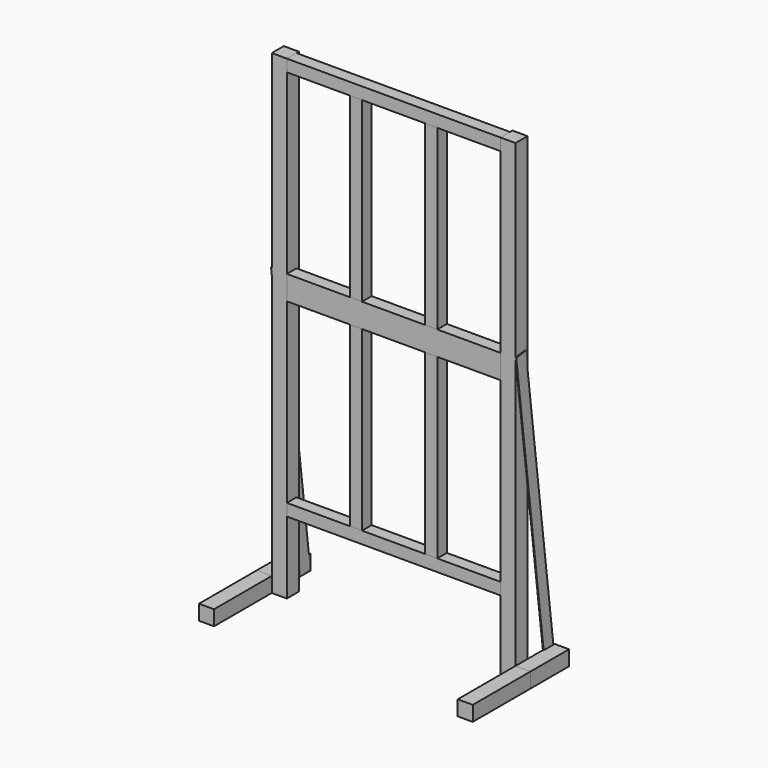
from build123d import *

# Parameters (mm, degrees)
F0_W      = 63.5
F0_H      = 63.5
F1_DEPTH  = 2006.6
F2_W      = 63.5
F2_H      = 63.5
F3_DEPTH  = 304.8
F4_DEPTH  = 203.2
F5_W      = 50.8
F5_H      = 50.8
F6_DEPTH  = 901.7
F7_W      = 50.8
F7_H      = 50.8
F8_DEPTH  = 749.3
F9_W      = 50.8
F9_H      = 50.8
F10_DEPTH = 749.3
F12_DEPTH = 3.175


# Not quite as in the source:
# - a length typed as a fraction of an inch, garbled in the dataset ("3 / 203.2 mm" for 3/8 in), is restored


with BuildPart() as f1:
    # F0 (on Top) → F1 (new body)
    with BuildSketch(Plane.XY):
        with Locations((-482.6, 31.75)):
            Rectangle(F0_W, F0_H)
    extrude(amount=F1_DEPTH)


with BuildPart() as f1b:
    # F0 (on Top) → F1, piece 2 (new body)
    with BuildSketch(Plane.XY):
        with Locations((482.6, 31.75)):
            Rectangle(F0_W, F0_H)
    extrude(amount=F1_DEPTH)


with BuildPart() as f3:
    # F2 (on Front) → F3 (new body)
    with BuildSketch(Plane.XZ):
        with Locations((-546.1, 31.75)):
            Rectangle(F2_W, F2_H)
    extrude(amount=F3_DEPTH)


with BuildPart() as f3b:
    # F2 (on Front) → F3, piece 2 (new body)
    with BuildSketch(Plane.XZ):
        with Locations((546.1, 31.75)):
            Rectangle(F2_W, F2_H)
    extrude(amount=F3_DEPTH)


with BuildPart() as f4:
    # F4 (new): a face of the model
    f4_faces = [f3.part.faces().sort_by_distance(p)[0] for p in [
        (-546.1, 0, 31.75),
    ]]
    extrude(f4_faces, amount=F4_DEPTH)


with BuildPart() as f4b:
    # F4#2 (new): a face of the model
    f4_2_faces = [f3b.part.faces().sort_by_distance(p)[0] for p in [
        (546.1, 0, 31.75),
    ]]
    extrude(f4_2_faces, amount=F4_DEPTH)


with BuildPart() as f6:
    # F5 (on face) → F6 (new body, through all)
    with BuildSketch(Plane.YZ.offset(-450.85)):
        with Locations((25.4, 1981.2)):
            Rectangle(F5_W, F5_H)
    extrude(amount=F6_DEPTH)


with BuildPart() as f6b:
    # F5 (on face) → F6, piece 2 (new body, through all)
    with BuildSketch(Plane.YZ.offset(-450.85)):
        with Locations((25.4, 1181.1)):
            Rectangle(F5_W, F5_H)
        with Locations((25.4, 1130.3)):
            Rectangle(F5_W, F5_H)
    extrude(amount=F6_DEPTH)


with BuildPart() as f6c:
    # F5 (on face) → F6, piece 3 (new body, through all)
    with BuildSketch(Plane.YZ.offset(-450.85)):
        with Locations((25.4, 330.2)):
            Rectangle(F5_W, F5_H)
    extrude(amount=F6_DEPTH)


with BuildPart() as f8:
    # F7 (on face) → F8 (new body, through all)
    with BuildSketch(Plane(origin=(0, 0, 1955.8), x_dir=(1, 0, 0), z_dir=(0, 0, -1))):
        with Locations((-158.75, -25.4)):
            Rectangle(F7_W, F7_H)
    extrude(amount=F8_DEPTH)


with BuildPart() as f8b:
    # F7 (on face) → F8, piece 2 (new body, through all)
    with BuildSketch(Plane(origin=(0, 0, 1955.8), x_dir=(1, 0, 0), z_dir=(0, 0, -1))):
        with Locations((158.75, -25.4)):
            Rectangle(F7_W, F7_H)
    extrude(amount=F8_DEPTH)


with BuildPart() as f10:
    # F9 (on face) → F10 (new body, through all)
    with BuildSketch(Plane(origin=(0, 0, 1104.9), x_dir=(1, 0, 0), z_dir=(0, 0, -1))):
        with Locations((158.75, -25.4)):
            Rectangle(F9_W, F9_H)
    extrude(amount=F10_DEPTH)


with BuildPart() as f10b:
    # F9 (on face) → F10, piece 2 (new body, through all)
    with BuildSketch(Plane(origin=(0, 0, 1104.9), x_dir=(1, 0, 0), z_dir=(0, 0, -1))):
        with Locations((-158.75, -25.4)):
            Rectangle(F9_W, F9_H)
    extrude(amount=F10_DEPTH)


with BuildPart() as f12:
    # F11 (on face) → F12 (new body)
    with BuildSketch(Plane(origin=(-514.35, 0, 0), x_dir=(0, -1, 0), z_dir=(-1, 0, 0))):
        Polygon((-63.5, 706.913542014), (-63.5, 1112.2482272862), (-203.2, 6.366689291), (-152.8005429844, 0), align=None)
        Polygon((0, 1209.5869683754), (-50.3994570156, 1215.9536576665), (-63.5, 1112.2482272862), (-63.5, 706.913542014), align=None)
    extrude(amount=F12_DEPTH)


with BuildPart() as f13_1:
    # F13: instance of F12
    add(f12.part.mirror(Plane.YZ))


solid = Compound([f1.part, f1b.part, f3.part, f3b.part, f4.part, f4b.part, f6.part, f6b.part, f6c.part, f8.part, f8b.part, f10.part, f10b.part, f12.part, f13_1.part])
